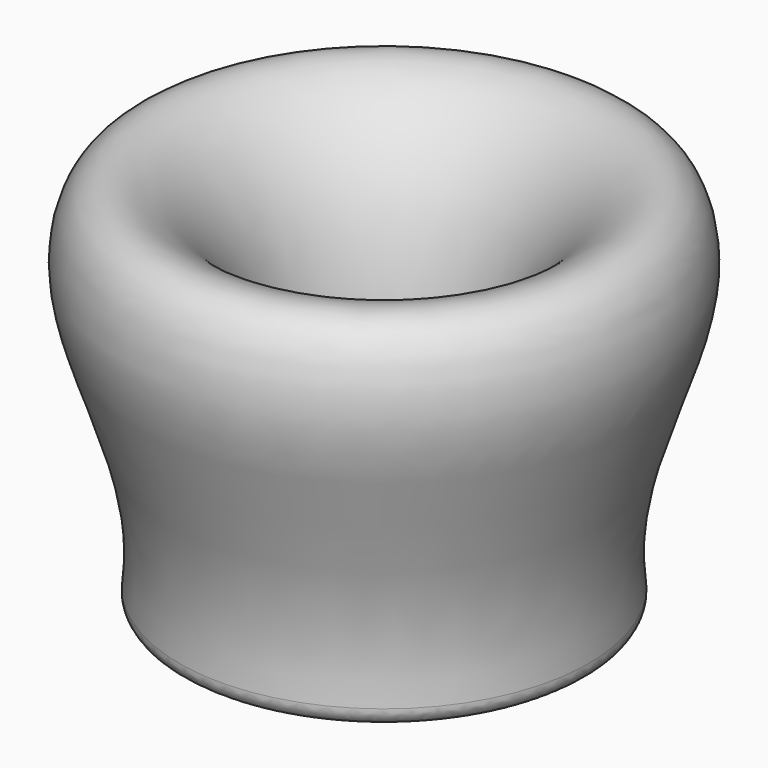
from build123d import *

# Parameters (mm, degrees)
F2_R = 5


with BuildPart() as f1:
    # F0 (on Front) → F1 (revolve)
    with BuildSketch(Plane.XZ):
        with BuildLine():
            add(Edge.make_bspline(
                [(-66.2219049335, 0), (-58.8383853396, 36.7197514066), (-92.9915691084, 84.9166402133), (-74.692706734, 131.4474340293), (-27.3414111183, 95.4728029291), (-30.9236581175, 38.028048283), (-31.2440937071, 0)],
                knots=[0, 0, 0, 0, 0.3097644403, 0.4857202638, 0.6836474525, 1, 1, 1, 1], degree=3))
            Line((-66.2219049335, 0), (-31.2440937071, 0))
        make_face()
    revolve(axis=Axis((0, 0, 57.1323619224), (0, 0, 1)))

    # F2
    f2_edges = [f1.edges().sort_by_distance(p)[0] for p in [
        (66.221905, 0, 0),
        (31.244094, 0, 0),
    ]]
    fillet(f2_edges, radius=F2_R)


solid = f1.part
